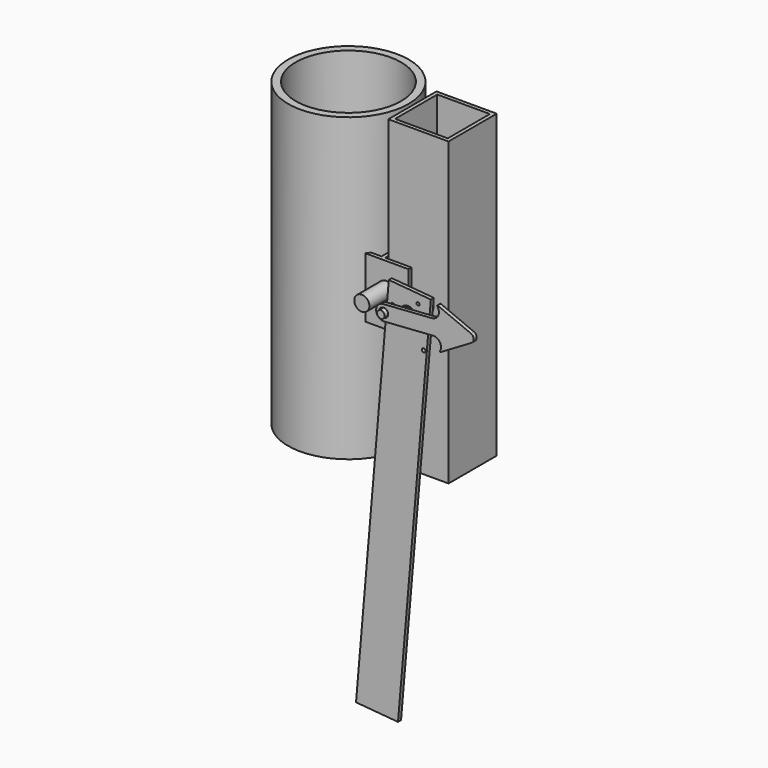
from build123d import *

# Parameters (mm, degrees)
F1_DEPTH  = 25.4
F2_R      = 3.175
F3_DEPTH  = 14.3202627102
F4_R      = 50.8
F4_R_2    = 44.45
F5_DEPTH  = 127
F4_W      = 50.8
F4_H      = 50.8
F4_W_2    = 44.45
F4_H_2    = 44.45
F6_R      = 6.35
F7_DEPTH  = 25.4
F8_R      = 6.35
F9_DEPTH  = 20.32
F11_START = 50.8
F10_R     = 3.81
F11_DEPTH = 3.175
F12_START = 15.875
F8_R_2    = 3.175
F8_R_3    = 6.477
F8_R_4    = 1.5494
F8_R_5    = 1.27
F12_DEPTH = 3.175
F13_START = 19.05
F13_DEPTH = 12.7


# Not quite as in the source:
# - a feature names something its author has since deleted; it is built from what else it names


with BuildPart() as f1:
    # F0 (on Top) → F1 (new body, symmetric)
    with BuildSketch(Plane.XY):
        with BuildLine():
            Line((0, 28.575), (0, 31.75))
            Line((0, 31.75), (-11.1442627102, 31.75))
            ThreePointArc((-11.1442627102, 31.75), (-9.940629285, 30.1852915304), (-8.7986979368, 28.575))
            Line((-8.7986979368, 28.575), (0, 28.575))
        make_face()
        Polygon((25.4, 28.575), (25.4, 31.75), (0, 31.75), (0, 28.575), (0, -28.575), (0, -31.75), (25.4, -31.75), (25.4, -28.575), (3.175, -28.575), (3.175, 28.575), align=None)
        with BuildLine():
            Line((0, -31.75), (0, -28.575))
            Line((0, -28.575), (-8.7986979368, -28.575))
            ThreePointArc((-8.7986979368, -28.575), (-9.940629285, -30.1852915304), (-11.1442627102, -31.75))
            Line((-11.1442627102, -31.75), (0, -31.75))
        make_face()
    extrude(amount=F1_DEPTH, both=True)

    # F2 (on face) → F3 (cut, through all)
    with BuildSketch(Plane.YZ.offset(3.175)):
        with Locations((0, 25.4)):
            Circle(F2_R)
    extrude(amount=-F3_DEPTH, mode=Mode.SUBTRACT)

    # F6 (on face) → F7 (join)
    with BuildSketch(Plane.XZ.offset(31.75)):
        with Locations((6.2447981909, 4.2749713175)):
            Circle(F6_R)
    extrude(amount=F7_DEPTH)


with BuildPart() as f5:
    # F4 (on Top) → F5 (new body, symmetric)
    with BuildSketch(Plane.XY):
        with Locations((-50.8, 0)):
            Circle(F4_R)
        with Locations((-50.8, 0)):
            Circle(F4_R_2, mode=Mode.SUBTRACT)
    extrude(amount=F5_DEPTH, both=True)


with BuildPart() as f5b:
    # F4 (on Top) → F5, piece 2 (new body, symmetric)
    with BuildSketch(Plane.XY):
        with Locations((28.575, 0)):
            Rectangle(F4_W, F4_H)
        with Locations((28.575, 0)):
            Rectangle(F4_W_2, F4_H_2, mode=Mode.SUBTRACT)
    extrude(amount=F5_DEPTH, both=True)

    # F8 (on face) → F9 (join)
    with BuildSketch(Plane.XZ.offset(25.4)):
        with Locations((34.925, 0)):
            Circle(F8_R)
    extrude(amount=F9_DEPTH)


with BuildPart() as f11:
    # F10 (on Front) → F11 (new body)
    with BuildSketch(Plane.XZ.offset(F11_START)):
        with BuildLine():
            Line((62.8270369727, 10.2701259875), (21.6521058039, 7.3977283401))
            ThreePointArc((21.6521058039, 7.3977283401), (15.759408339, 0.6212162145), (22.5359204646, -5.2714812503))
            Line((22.5359204646, -5.2714812503), (63.7108516334, -2.3990836029))
            ThreePointArc((63.7108516334, -2.3990836029), (69.5933796071, -5.4592194313), (69.5433316896, -12.0899103346))
            ThreePointArc((69.5433316896, -12.0899103346), (69.5942249576, -12.5575210472), (70.0605169279, -12.6193409606))
            Line((70.0605169279, -12.6193409606), (96.1969817693, 2.8168733057))
            ThreePointArc((96.1969817693, 2.8168733057), (98.0602358988, 6.3625908021), (95.7227206874, 9.6152591148))
            Line((95.7227206874, 9.6152591148), (67.6961578025, 21.2730152514))
            ThreePointArc((67.6961578025, 21.2730152514), (67.2429657872, 21.1470513659), (67.2574913344, 20.6769036107))
            ThreePointArc((67.2574913344, 20.6769036107), (68.2276991914, 14.1173866037), (62.8270369727, 10.2701259875))
        make_face()
        with Locations((22.0940131342, 1.0631235449)):
            Circle(F10_R, mode=Mode.SUBTRACT)
    extrude(amount=F11_DEPTH)


with BuildPart() as f12:
    # F8 (on face) → F12 (new body)
    with BuildSketch(Plane.XZ.offset(25.4).offset(F12_START)):
        Polygon((18.8372476626, 20.499149366), (-8.8261978146, -302.1671740772), (26.6038298576, -305.2047288747), (54.2672753347, 17.4615945685), align=None)
        with Locations((22.2714186885, 1.0848409991)):
            Circle(F8_R_2, mode=Mode.SUBTRACT)
        with Locations((34.925, 0)):
            Circle(F8_R_3, mode=Mode.SUBTRACT)
        with Locations((48.1789697316, -22.2411817218)):
            Circle(F8_R_4, mode=Mode.SUBTRACT)
        with Locations((43.4935056861, 10.7373185809)):
            Circle(F8_R_5, mode=Mode.SUBTRACT)
        with Locations((22.2714186885, 1.0848409991)):
            Circle(F8_R_2)
    extrude(amount=F12_DEPTH)

    # F8 (on face) → F13 (join)
    with BuildSketch(Plane.XZ.offset(25.4).offset(F13_START)):
        with Locations((22.2714186885, 1.0848409991)):
            Circle(F8_R_2)
    extrude(amount=F13_DEPTH)


solid = Compound([f1.part, f5.part, f5b.part, f11.part, f12.part])
